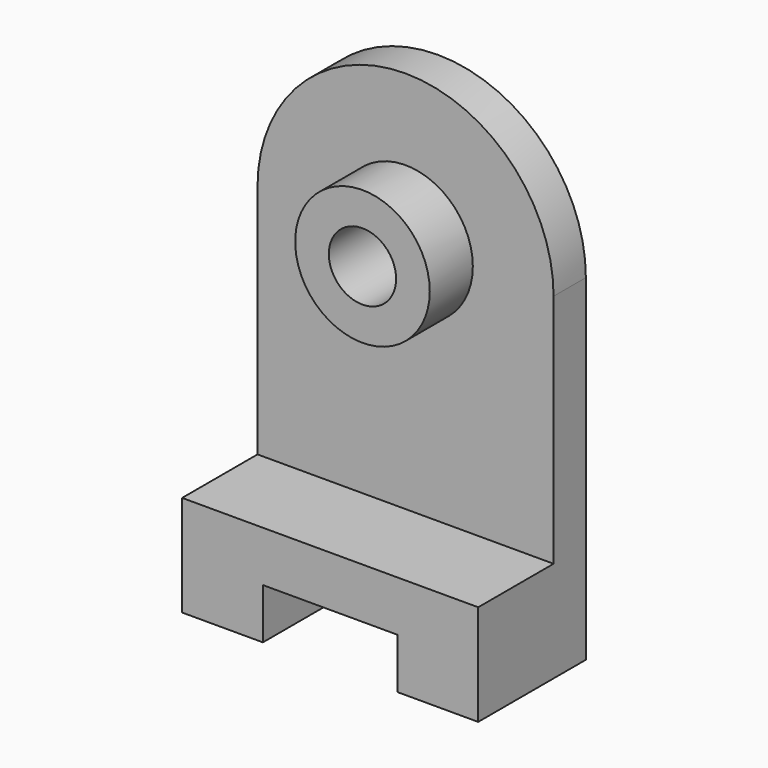
from build123d import *

# Parameters (mm, degrees)
F0_R     = 20
F0_R_2   = 10
F1_DEPTH = 28
F2_DEPTH = 12
F3_DEPTH = 40


# Not quite as in the source:
# - ends of sketch curves that miss each other by under 0.0002 mm in the source are joined


with BuildPart() as f1:
    # F0 (on Front) → F1 (new body)
    with BuildSketch(Plane.XZ):
        with Locations((0, 32)):
            Circle(F0_R)
        with Locations((0, 32)):
            Circle(F0_R_2, mode=Mode.SUBTRACT)
    extrude(amount=F1_DEPTH)

    # F0 (on Front) → F2 (join)
    with BuildSketch(Plane.XZ):
        with BuildLine():
            add(Edge.make_bspline(
                [(-43.9999970173, -38), (-43.9999970173, -14.6666666667), (-43.9999970173, 8.6666666667), (-43.9999970173, 32)],
                knots=[0, 0, 0, 0, 70, 70, 70, 70], degree=3))
            Line((-43.9999970173, -38), (44, -38))
            Line((44, -38), (44, 32))
            ThreePointArc((44, 32), (0, 76), (-43.9999970173, 32))
        make_face()
        with Locations((0, 32)):
            Circle(F0_R, mode=Mode.SUBTRACT)
    extrude(amount=F2_DEPTH)

    # F0 (on Front) → F3 (join)
    with BuildSketch(Plane.XZ):
        Polygon((-43.9999970173, -38), (-43.9999970173, -68), (-20, -68), (-20, -53), (20, -53), (20, -68), (44, -68), (44, -38), align=None)
    extrude(amount=F3_DEPTH)


solid = f1.part
